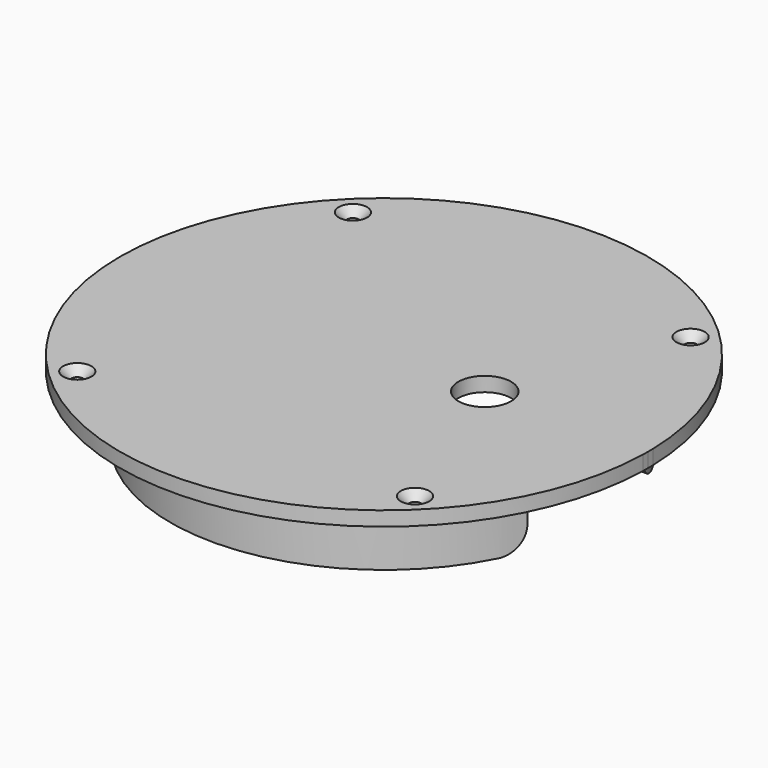
from build123d import *

# Parameters (mm, degrees)
F0_R        = 1.25
F0_R_2      = 5.5
F1_DEPTH    = 3
F3_DEPTH    = 13.4
F4_T1_DEPTH = 26.5968204778
F5_SIZE     = 1.7


# Not quite as in the source:
# - a fillet or chamfer that OpenCascade refuses, or shapes differently, is made with other operations: its cross-section is extruded or revolved along the edge and cut away or added
# - a feature names something its author has since deleted; it is built from what else it names


with BuildPart() as f1:
    # F0 (on Top) → F1 (new body)
    with BuildSketch(Plane.XY):
        with BuildLine():
            ThreePointArc((45.3208194724, 4.0340206186), (-45.5, 0), (45.3208194724, -4.0340206186))
            ThreePointArc((45.3208194724, -4.0340206186), (46.2839051451, -2.086638513), (48.3090053717, -1.3))
            Line((48.3090053717, -1.3), (54.9846342172, -1.3))
            ThreePointArc((54.9846342172, -1.3), (54.9961584201, -0.6500454037), (55, 0))
            ThreePointArc((55, 0), (54.9961584201, 0.6500454037), (54.9846342172, 1.3))
            Line((54.9846342172, 1.3), (48.3090053717, 1.3))
            ThreePointArc((48.3090053717, 1.3), (46.2839051451, 2.086638513), (45.3208194724, 4.0340206186))
        make_face()
        with BuildLine():
            Line((39.2652518138, 1.3), (32, 1.3))
            Line((32, 1.3), (32, 0))
            Line((32, 0), (32, -1.3))
            Line((32, -1.3), (39.2652518138, -1.3))
            ThreePointArc((39.2652518138, -1.3), (41.499054271, -2.2974699547), (42.2474228376, -4.6265822785))
            ThreePointArc((42.2474228376, -4.6265822785), (-42.5, 0), (42.2474228376, 4.6265822785))
            ThreePointArc((42.2474228376, 4.6265822785), (41.499054271, 2.2974699547), (39.2652518138, 1.3))
        make_face(mode=Mode.SUBTRACT)
        with BuildLine():
            Line((32, 15), (32, 1.3))
            Line((32, 1.3), (39.2652518138, 1.3))
            ThreePointArc((39.2652518138, 1.3), (41.499054271, 2.2974699547), (42.2474228376, 4.6265822785))
            ThreePointArc((42.2474228376, 4.6265822785), (-42.5, 0), (42.2474228376, -4.6265822785))
            ThreePointArc((42.2474228376, -4.6265822785), (41.499054271, -2.2974699547), (39.2652518138, -1.3))
            Line((39.2652518138, -1.3), (32, -1.3))
            Line((32, -1.3), (32, -15))
            Line((32, -15), (21.575, -15))
            Line((21.575, -15), (21.575, -17.3))
            ThreePointArc((21.575, -17.3), (17.075, -21.8), (12.575, -17.3))
            Line((12.575, -17.3), (12.575, -15))
            Line((12.575, -15), (-12.575, -15))
            Line((-12.575, -15), (-12.575, -17.3))
            ThreePointArc((-12.575, -17.3), (-17.075, -21.8), (-21.575, -17.3))
            Line((-21.575, -17.3), (-21.575, -15))
            Line((-21.575, -15), (-32, -15))
            Line((-32, -15), (-32, 15))
            Line((-32, 15), (-21.575, 15))
            Line((-21.575, 15), (-21.575, 17.3))
            ThreePointArc((-21.575, 17.3), (-17.075, 21.8), (-12.575, 17.3))
            Line((-12.575, 17.3), (-12.575, 15))
            Line((-12.575, 15), (12.575, 15))
            Line((12.575, 15), (12.575, 17.3))
            ThreePointArc((12.575, 17.3), (17.075, 21.8), (21.575, 17.3))
            Line((21.575, 17.3), (21.575, 15))
            Line((21.575, 15), (32, 15))
        make_face()
        with BuildLine():
            ThreePointArc((48.3090053717, -1.3), (46.2839051451, -2.086638513), (45.3208194724, -4.0340206186))
            ThreePointArc((45.3208194724, -4.0340206186), (-45.5, 0), (45.3208194724, 4.0340206186))
            ThreePointArc((45.3208194724, 4.0340206186), (46.2839051451, 2.086638513), (48.3090053717, 1.3))
            Line((48.3090053717, 1.3), (54.9846342172, 1.3))
            ThreePointArc((54.9846342172, 1.3), (-55, 0), (54.9846342172, -1.3))
            Line((54.9846342172, -1.3), (48.3090053717, -1.3))
        make_face()
        with Locations((-35.175, -35.8856778534)):
            Circle(F0_R, mode=Mode.SUBTRACT)
        with Locations((35.175, -35.8856778534)):
            Circle(F0_R, mode=Mode.SUBTRACT)
        with Locations((-35.175, 35.8856778534)):
            Circle(F0_R, mode=Mode.SUBTRACT)
        with Locations((35.175, 35.8856778534)):
            Circle(F0_R, mode=Mode.SUBTRACT)
        with BuildLine():
            Line((32, 0), (32, 1.3))
            Line((32, 1.3), (32, 15))
            Line((32, 15), (21.575, 15))
            Line((21.575, 15), (21.575, 17.3))
            ThreePointArc((21.575, 17.3), (17.075, 21.8), (12.575, 17.3))
            Line((12.575, 17.3), (12.575, 15))
            Line((12.575, 15), (-12.575, 15))
            Line((-12.575, 15), (-12.575, 17.3))
            ThreePointArc((-12.575, 17.3), (-17.075, 21.8), (-21.575, 17.3))
            Line((-21.575, 17.3), (-21.575, 15))
            Line((-21.575, 15), (-32, 15))
            Line((-32, 15), (-32, -15))
            Line((-32, -15), (-21.575, -15))
            Line((-21.575, -15), (-21.575, -17.3))
            ThreePointArc((-21.575, -17.3), (-17.075, -21.8), (-12.575, -17.3))
            Line((-12.575, -17.3), (-12.575, -15))
            Line((-12.575, -15), (12.575, -15))
            Line((12.575, -15), (12.575, -17.3))
            ThreePointArc((12.575, -17.3), (17.075, -21.8), (21.575, -17.3))
            Line((21.575, -17.3), (21.575, -15))
            Line((21.575, -15), (32, -15))
            Line((32, -15), (32, -1.3))
            Line((32, -1.3), (32, 0))
        make_face()
        with Locations((21, 0)):
            Circle(F0_R_2, mode=Mode.SUBTRACT)
    extrude(amount=F1_DEPTH)

    # F2 (on face) → F3 (join)
    with BuildSketch(Plane(origin=(0, 0, 0), x_dir=(1, 0, 0), z_dir=(0, 0, -1))):
        with BuildLine():
            Line((40.2988833592, 15), (41.895703837, 15))
            ThreePointArc((41.895703837, 15), (-44.5, 0), (41.895703837, -15))
            Line((41.895703837, -15), (40.2988833592, -15))
            ThreePointArc((40.2988833592, -15), (-43, 0), (40.2988833592, 15))
        make_face()
    extrude(amount=F3_DEPTH)

    # F4: fillet of radius 5 on 2 edges, made by hand

    # F4_s2 → F4_t1 (cut)
    with BuildSketch(Plane.YZ.offset(27.7988833592)):
        with BuildLine():
            ThreePointArc((-15, -8.4), (-16.4644660941, -11.9355339059), (-20, -13.4))
            Line((-20, -13.4), (-15, -13.4))
            Line((-15, -13.4), (-15, -8.4))
        make_face()
        with BuildLine():
            ThreePointArc((15, -8.4), (16.4644660941, -11.9355339059), (20, -13.4))
            Line((20, -13.4), (15, -13.4))
            Line((15, -13.4), (15, -8.4))
        make_face()
    extrude(amount=F4_T1_DEPTH, mode=Mode.SUBTRACT)

    # F5
    f5_edges = [f1.edges().sort_by_distance(p)[0] for p in [
        (-36.425, 35.885678, 3),
        (-36.425, -35.885678, 3),
        (33.925, -35.885678, 3),
        (33.925, 35.885678, 3),
    ]]
    chamfer(f5_edges, length=F5_SIZE)


solid = f1.part
